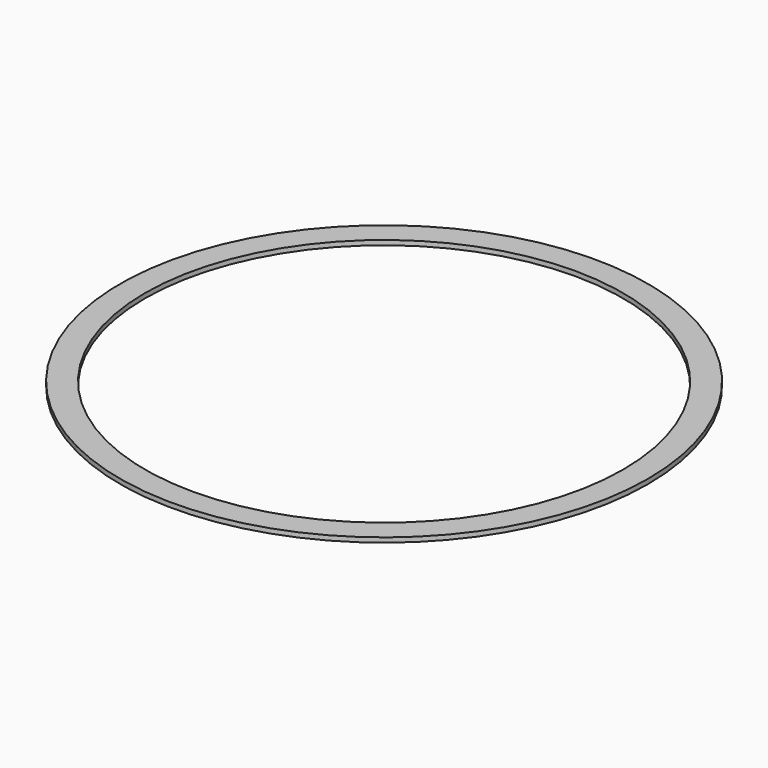
from build123d import *

# Parameters (mm, degrees)
F0_R     = 269.05331
F0_R_2   = 243.65331
F1_DEPTH = 4.7625


# Not quite as in the source:
# - a length typed as a fraction of an inch, garbled in the dataset ("3 / 203.2 mm" for 3/8 in), is restored


with BuildPart() as f1:
    # F0 (on Top) → F1 (new body)
    with BuildSketch(Plane.XY):
        Circle(F0_R)
        Circle(F0_R_2, mode=Mode.SUBTRACT)
    extrude(amount=F1_DEPTH)


solid = f1.part
